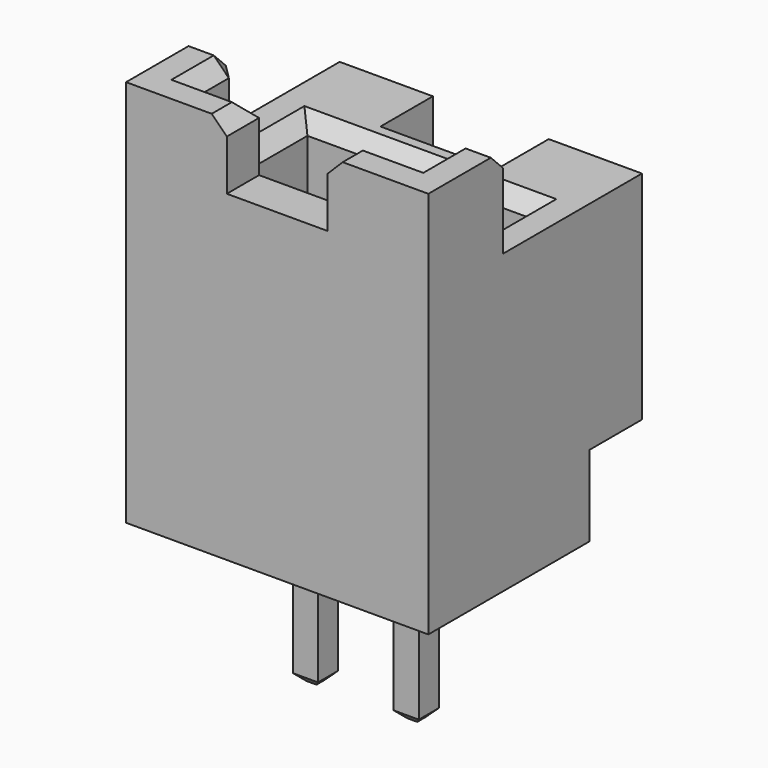
from build123d import *

# Parameters (mm, degrees)
F0_W          = 0.5
F0_H          = 0.5
F1_DEPTH      = 3
F1_DEPTH_BACK = 4
F2_W          = 6
F2_H          = 5.3
F3_DEPTH      = 7.7
F4_W          = 4.4
F4_H          = 2.7
F5_DEPTH      = 5.8
F6_W          = 2
F6_H          = 0.8
F7_DEPTH      = 1.3
F8_DEPTH      = 1.8
F9_W          = 2.3
F9_H          = 1.3
F10_DEPTH     = 25
F11_W         = 0.8
F11_H         = 1.84
F12_DEPTH     = 0.6
F13_W         = 1.85
F13_H         = 1.3
F14_DEPTH     = 1.6
F15_SIZE2     = 1
F15_SIZE      = 0.5
F16_SIZE      = 0.3
F17_SIZE      = 0.15
F17_2_SIZE    = 0.15


with BuildPart() as f1:
    # F0 (on Top) → F1 (new body, two sides)
    with BuildSketch(Plane.XY) as f1_sk:
        with Locations((-2, 0)):
            Rectangle(F0_W, F0_H)
    extrude(amount=-F1_DEPTH)
    extrude(f1_sk.sketch, amount=F1_DEPTH_BACK)

    # F17
    f17_edges = [f1.edges().sort_by_distance(p)[0] for p in [
        (-2, 0.25, 4),
        (-2.25, 0, 4),
        (-2, -0.25, 4),
        (-1.75, 0, 4),
        (-2, 0.25, -3),
        (-2.25, 0, -3),
        (-2, -0.25, -3),
        (-1.75, 0, -3),
    ]]
    chamfer(f17_edges, length=F17_SIZE)


with BuildPart() as f1b:
    # F0 (on Top) → F1, piece 2 (new body, two sides)
    with BuildSketch(Plane.XY) as f1_2_sk:
        Rectangle(F0_W, F0_H)
    extrude(amount=-F1_DEPTH)
    extrude(f1_2_sk.sketch, amount=F1_DEPTH_BACK)

    # F17#2
    f17_2_edges = [f1b.edges().sort_by_distance(p)[0] for p in [
        (0.25, 0, 4),
        (0, 0.25, 4),
        (-0.25, 0, 4),
        (0, -0.25, 4),
        (0.25, 0, -3),
        (0, 0.25, -3),
        (-0.25, 0, -3),
        (0, -0.25, -3),
    ]]
    chamfer(f17_2_edges, length=F17_2_SIZE)


with BuildPart() as f3:
    # F2 (on Top) → F3 (new body)
    with BuildSketch(Plane.XY):
        with Locations((-1, 0.45)):
            Rectangle(F2_W, F2_H)
    extrude(amount=F3_DEPTH)

    # F4 (on face) → F5 (cut)
    with BuildSketch(Plane.XY.offset(7.7)):
        with Locations((-1, -0.05)):
            Rectangle(F4_W, F4_H)
    extrude(amount=-F5_DEPTH, mode=Mode.SUBTRACT)

    # F6 (on face) → F7 (cut)
    with BuildSketch(Plane.XY.offset(7.7)):
        with Locations((-1, -1.8)):
            Rectangle(F6_W, F6_H)
    extrude(amount=-F7_DEPTH, mode=Mode.SUBTRACT)

    # F6 (on face) → F8 (cut)
    with BuildSketch(Plane.XY.offset(7.7)):
        Polygon((-4, 3.1), (-4, -0.35), (-3.2, -0.35), (-3.2, 1.3), (1.2, 1.3), (1.2, -0.35), (2, -0.35), (2, 3.1), align=None)
    extrude(amount=-F8_DEPTH, mode=Mode.SUBTRACT)

    # F9 (on face) → F10 (cut)
    with BuildSketch(Plane.XY.offset(5.9)):
        with Locations((-1, 2.45)):
            Rectangle(F9_W, F9_H)
    extrude(amount=-F10_DEPTH, mode=Mode.SUBTRACT)

    # F11 (on face) → F12 (join)
    with BuildSketch(Plane(origin=(0, 1.8, 0), x_dir=(-1, 0, 0), z_dir=(0, 1, 0))):
        with Locations((1, 4.02)):
            Rectangle(F11_W, F11_H)
    extrude(amount=F12_DEPTH)

    # F13 (on face) → F14 (cut)
    with BuildSketch(Plane(origin=(0, 0, 0), x_dir=(1, 0, 0), z_dir=(0, 0, -1))):
        with Locations((-3.075, -2.45)):
            Rectangle(F13_W, F13_H)
        with Locations((1.075, -2.45)):
            Rectangle(F13_W, F13_H)
    extrude(amount=-F14_DEPTH, mode=Mode.SUBTRACT)

    # F15
    f15_edges = [f3.edges().sort_by_distance(p)[0] for p in [
        (-1, 2.4, 4.94),
    ]]
    f15_side = f3.faces().sort_by_distance((-1, 2.1, 4.94))[0]
    chamfer(f15_edges, length=F15_SIZE, length2=F15_SIZE2, reference=f15_side)

    # F16
    f16_edges = [f3.edges().sort_by_distance(p)[0] for p in [
        (-2.6, -1.4, 7.7),
        (-3.2, -0.875, 7.7),
        (0.6, -1.4, 7.7),
        (1.2, -0.875, 7.7),
        (-2, -1.8, 7.7),
        (0, -1.8, 7.7),
        (-3.6, -0.35, 7.7),
        (1.6, -0.35, 7.7),
        (1.2, -0.35, 6.8),
        (1.2, 0.475, 5.9),
        (-1, 1.3, 5.9),
        (-3.2, 0.475, 5.9),
        (-3.2, -0.35, 6.8),
    ]]
    chamfer(f16_edges, length=F16_SIZE)


solid = Compound([f1.part, f1b.part, f3.part])
